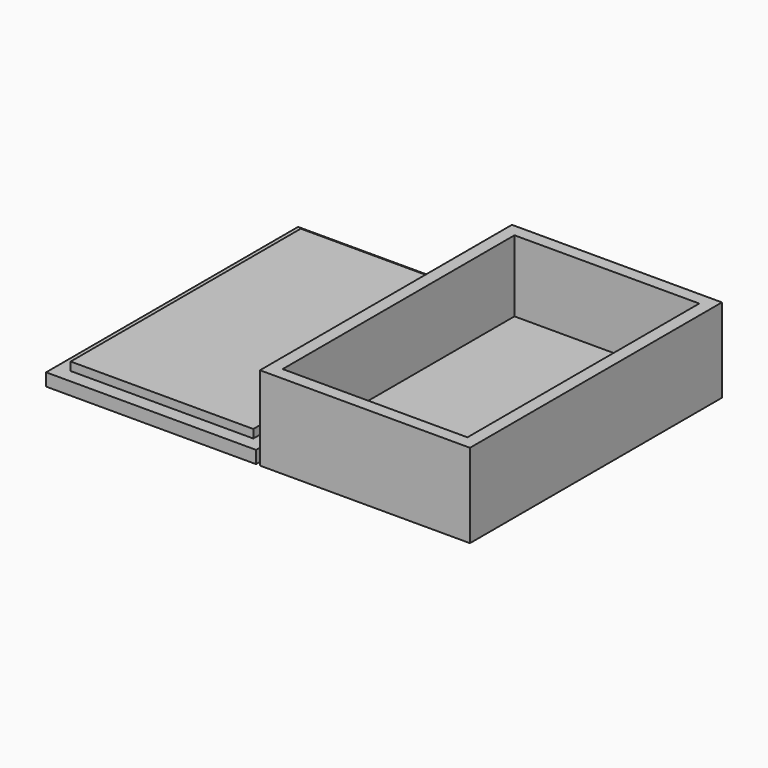
from build123d import *

# Parameters (mm, degrees)
F0_W         = 50
F0_H         = 75
F1_DEPTH     = 20
F2_W         = 44
F2_H         = 69
F3_DEPTH     = 17
F4_W         = 50
F4_H         = 75
F5_DEPTH     = 3
F6_W         = 43.5
F6_H         = 68.5
F7_DEPTH     = 2
F8_TEXT_SIZE = 17.2167085111
F9_DEPTH     = 2


# Not quite as in the source:
# - Text() gives the source's letters only with a copy of the font that has no kerning and outlines rounded to 1/6400 em; it was checked with that copy


with BuildPart() as f1:
    # F0 (on Top) → F1 (new body)
    with BuildSketch(Plane.XY):
        with Locations((25, 37.5)):
            Rectangle(F0_W, F0_H)
    extrude(amount=F1_DEPTH)

    # F2 (on face) → F3 (cut)
    with BuildSketch(Plane.XY.offset(20)):
        with Locations((25, 37.5)):
            Rectangle(F2_W, F2_H)
    extrude(amount=-F3_DEPTH, mode=Mode.SUBTRACT)


with BuildPart() as f5:
    # F4 (on Top) → F5 (new body)
    with BuildSketch(Plane.XY):
        with Locations((-25.9370788932, 37.5)):
            Rectangle(F4_W, F4_H)
    extrude(amount=F5_DEPTH)

    # F6 (on face) → F7 (join)
    with BuildSketch(Plane.XY.offset(3)):
        with Locations((-25.9370788932, 37.5)):
            Rectangle(F6_W, F6_H)
    extrude(amount=F7_DEPTH)

    # F8 (on face) → F9 (cut)
    with BuildSketch(Plane(origin=(0, 0, 0), x_dir=(1, 0, 0), z_dir=(0, 0, -1))):
        with Locations(Location((-20.9243891761, -62.515027108), (0, 0, 90))):
            Text('Janice', F8_TEXT_SIZE, font='Open Sans', text_align=(TextAlign.LEFT, TextAlign.BOTTOM))
    extrude(amount=-F9_DEPTH, mode=Mode.SUBTRACT)


solid = Compound([f1.part, f5.part])
